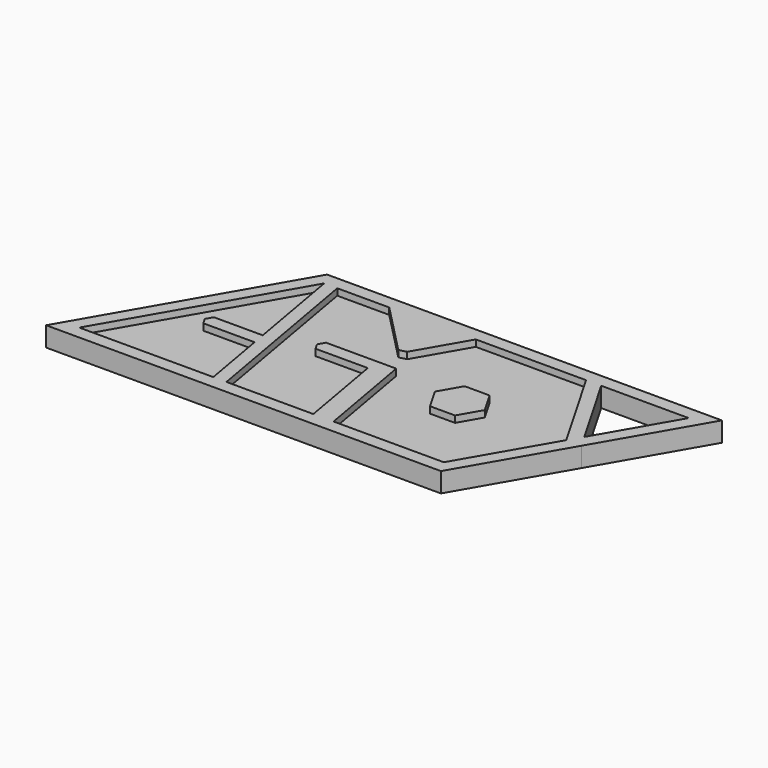
from build123d import *

# Parameters (mm, degrees)
F1_DEPTH = 2
F2_DEPTH = 3
F3_DEPTH = 3


# Not quite as in the source:
# - a feature names something its author has since deleted; it is built from what else it names


with BuildPart() as f1:
    # F0 (on Top) → F1 (new body)
    with BuildSketch(Plane.XY):
        Polygon((-43.2085677565, 22.6745967576), (-58.8549531333, -4.4257376699), (-38.4300476107, -4.4257376699), (-40.2088151152, 5.6621541398), (-48.0090622621, 5.6621541398), (-48.5864125313, 6.6621541398), (-48.0090622621, 7.6621541398), (-40.5614690766, 7.6621541398), align=None)
    extrude(amount=F1_DEPTH)



with BuildPart() as f1b:
    # F0 (on Top) → F1, piece 2 (new body)
    with BuildSketch(Plane.XY):
        Polygon((-41.2085677565, 22.6745967576), (-36.4300476107, -4.4257376699), (-25.5239465254, -4.4257376699), (-23.5239465254, -4.4257376699), (-23.1770010553, -4.4257376699), (-25.5239465254, 8.8844515061), (-33.4898163741, 8.8844515061), (-34.0671666433, 9.8844515061), (-33.4898163741, 10.8844515061), (-22.7936475677, 10.8844515061), (-20.0940481363, -4.4257376699), (-3.2846095154, -4.4257376699), (4.538583173, 9.1244295439), (-3.2846095154, 22.6745967576), (-20.0940481363, 22.6745967576), (-24.4790815038, 15.0794961721), (-25.6024042349, 14.7936511306), (-33.2868439501, 22.6745967576), align=None)
        Polygon((-15.4996355878, 9.1244295439), (-13.5944822068, 12.424251996), (-9.7841754448, 12.424251996), (-7.8790220638, 9.1244295439), (-9.7841754448, 5.8246070917), (-13.5944822068, 5.8246070917), align=None, mode=Mode.SUBTRACT)
    extrude(amount=F1_DEPTH)


with BuildPart() as f1_1:
    add(f1.part)

    add(f1b.part)  # F2 merges F1b
    # F0 (on Top) → F2 (join)
    with BuildSketch(Plane.XY):
        Polygon((-2.8602079346, 24.6745967576), (-44.3632682949, 24.6745967576), (-62.3190547484, -6.4257376699), (-38.9180315569, -6.4257376699), (-2.129908977, -6.4257376699), (6.8479842498, 9.1244295439), (15.8258774766, 24.6745967576), align=None)
        Polygon((-38.4300476107, -4.4257376699), (-58.8549531333, -4.4257376699), (-43.2085677565, 22.6745967576), (-41.2085677565, 22.6745967576), (-33.2868439501, 22.6745967576), (-30.5356123181, 22.6745967576), (-20.0940481363, 22.6745967576), (-3.2846095154, 22.6745967576), (4.538583173, 9.1244295439), (-3.2846095154, -4.4257376699), (-20.0940481363, -4.4257376699), (-23.1770010553, -4.4257376699), (-23.5239465254, -4.4257376699), (-25.5239465254, -4.4257376699), (-36.4300476107, -4.4257376699), align=None, mode=Mode.SUBTRACT)
        Polygon((12.3617758614, 22.6745967576), (5.6932837114, 11.1244295439), (-0.9752084386, 22.6745967576), align=None, mode=Mode.SUBTRACT)
        Polygon((-25.5239465254, 8.8844515061), (-23.1770010553, -4.4257376699), (-20.0940481363, -4.4257376699), (-22.7936475677, 10.8844515061), (-33.4898163741, 10.8844515061), (-34.0671666433, 9.8844515061), (-33.4898163741, 8.8844515061), align=None)
        Polygon((-40.2088151152, 5.6621541398), (-38.4300476107, -4.4257376699), (-36.4300476107, -4.4257376699), (-41.2085677565, 22.6745967576), (-43.2085677565, 22.6745967576), (-40.5614690766, 7.6621541398), align=None)
        Polygon((-20.0940481363, 22.6745967576), (-30.5356123181, 22.6745967576), (-24.1704509766, 16.1898996279), (-24.4790815038, 15.0794961721), align=None)
        Polygon((-30.5356123181, 22.6745967576), (-33.2868439501, 22.6745967576), (-25.6024042349, 14.7936511306), (-24.4790815038, 15.0794961721), (-24.1704509766, 16.1898996279), align=None)
        Polygon((-48.0090622621, 5.6621541398), (-40.2088151152, 5.6621541398), (-40.5614690766, 7.6621541398), (-48.0090622621, 7.6621541398), (-48.5864125313, 6.6621541398), align=None)
    extrude(amount=F2_DEPTH)

    # F0 (on Top) → F3 (join)
    with BuildSketch(Plane.XY):
        Polygon((-9.7841754448, 12.424251996), (-13.5944822068, 12.424251996), (-15.4996355878, 9.1244295439), (-13.5944822068, 5.8246070917), (-9.7841754448, 5.8246070917), (-7.8790220638, 9.1244295439), align=None)
    extrude(amount=F3_DEPTH)


solid = f1_1.part
